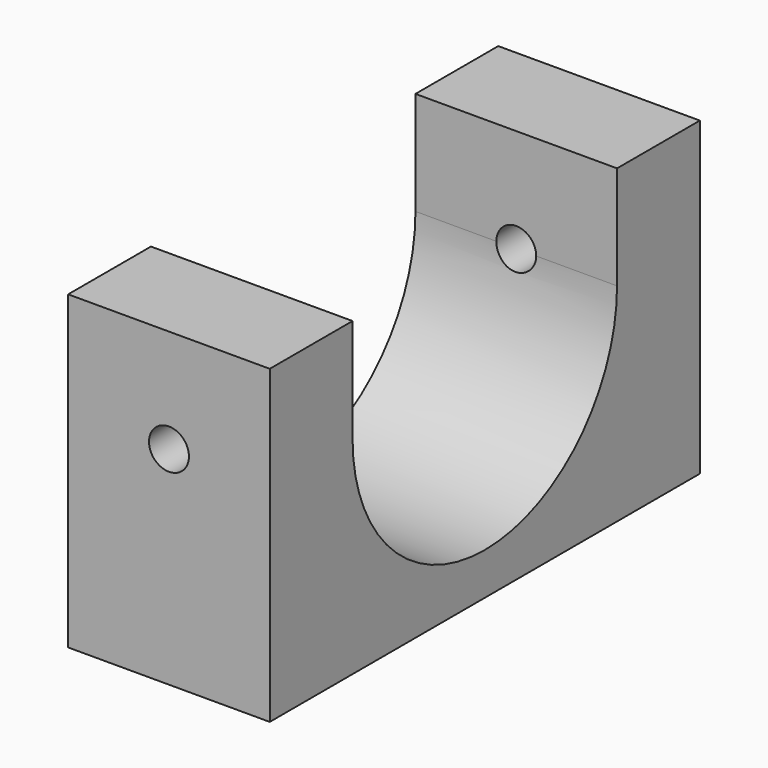
from build123d import *

# Parameters (mm, degrees)
F1_DEPTH = 19.05
F3_D     = 7.5438
F3_DEPTH = 25.4
F3_TIP   = 2.2663861689


# Not quite as in the source:
# - a pattern or mirror of a feature is missing from the dataset's text; its kind, count and spacing are read off the source's solid


with BuildPart() as f1:
    # F0 (on Right) → F1 (new body, symmetric)
    with BuildSketch(Plane.YZ):
        with BuildLine():
            Line((31.242, 19.558), (31.242, 0))
            ThreePointArc((31.242, 0), (0, -31.242), (-31.242, 0))
            Line((-31.242, 0), (-31.242, 19.558))
            Line((-31.242, 19.558), (-50.8, 19.558))
            Line((-50.8, 19.558), (-50.8, -39.1922))
            Line((-50.8, -39.1922), (0, -39.1922))
            Line((0, -39.1922), (50.8, -39.1922))
            Line((50.8, -39.1922), (50.8, 19.558))
            Line((50.8, 19.558), (31.242, 19.558))
        make_face()
    extrude(amount=F1_DEPTH, both=True)

    # F3
    with Locations(Plane(origin=(0, 50.8, 0), x_dir=(-1, 0, 0), z_dir=(0, 1, 0))):
        with Locations((0, 0)):
            f3 = Hole(F3_D / 2, depth=F3_DEPTH)
            with Locations((0, 0, -(F3_DEPTH + F3_TIP / 2))):  # 118° drill point
                Cone(0, F3_D / 2, F3_TIP, mode=Mode.SUBTRACT)

    # F3_copies: F3 across plane
    add(f3.mirror(Plane(origin=(0, 0, 0), x_dir=(0, 0, -1), z_dir=(0, -1, 0))), mode=Mode.SUBTRACT)


solid = f1.part
